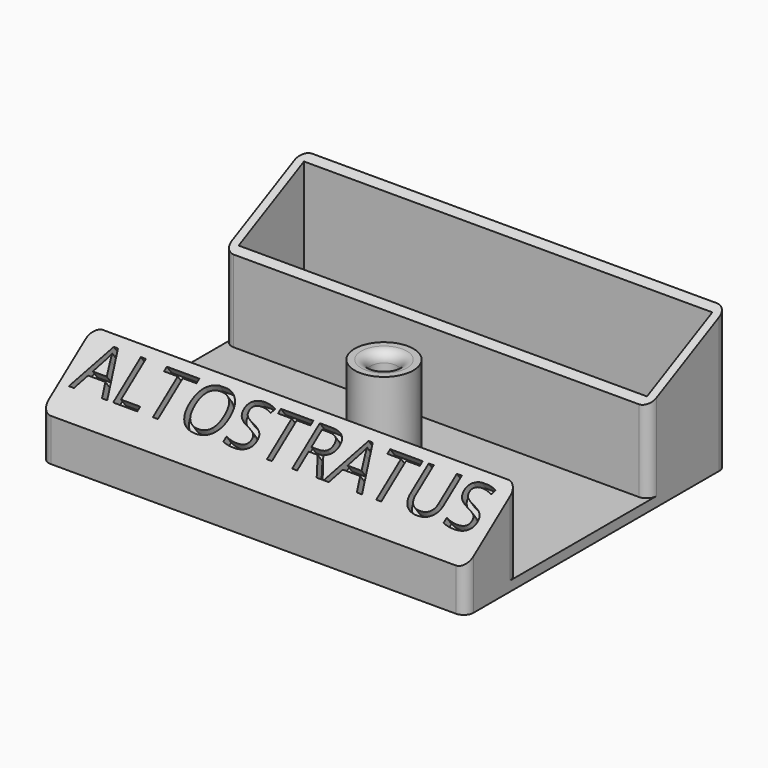
from build123d import *

# Parameters (mm, degrees)
F0_W        = 130
F0_H        = 100
F1_DEPTH    = 3
F2_W        = 130
F2_H        = 30
F2_W_2      = 125
F2_H_2      = 25
F3_DEPTH    = 40
F2_R        = 9
F2_R_2      = 4
F2_H_3      = 20
F4_DEPTH    = 25
F5_T1_DEPTH = 233.2279032045
F6_T1_DEPTH = 285.3897324272
F7_R        = 3
F9_DEPTH    = 3


# Not quite as in the source:
# - a fillet or chamfer that OpenCascade refuses, or shapes differently, is made with other operations: its cross-section is extruded or revolved along the edge and cut away or added


with BuildPart() as f1:
    # F0 (on Top) → F1 (new body)
    with BuildSketch(Plane.XY):
        with Locations((0, 50)):
            Rectangle(F0_W, F0_H)
    extrude(amount=F1_DEPTH)

    # F2 (on face) → F3 (join)
    with BuildSketch(Plane.XY.offset(3)):
        with Locations((0, 85)):
            Rectangle(F2_W, F2_H)
        with Locations((0, 85)):
            Rectangle(F2_W_2, F2_H_2, mode=Mode.SUBTRACT)
    extrude(amount=F3_DEPTH)

    # F2 (on face) → F4 (join)
    with BuildSketch(Plane.XY.offset(3)):
        with Locations((0, 50)):
            Circle(F2_R)
        with Locations((0, 50)):
            Circle(F2_R_2, mode=Mode.SUBTRACT)
        with Locations((0, 10)):
            Rectangle(F2_W, F2_H_3)
    extrude(amount=F4_DEPTH)

    # F5: chamfer of 20 x 15 on 1 edges, made by hand

    # F5_s2 → F5_t1 (cut)
    with BuildSketch(Plane.YZ.offset(-116.6139516023)):
        Polygon((0, 13), (20, 28), (0, 28), align=None)
    extrude(amount=F5_T1_DEPTH, mode=Mode.SUBTRACT)

    # F6: chamfer of 30 x 15 on 1 edges, made by hand

    # F6_s2 → F6_t1 (cut)
    with BuildSketch(Plane.YZ.offset(-142.6948662136)):
        Polygon((100, 43), (70, 28), (70, 43), align=None)
    extrude(amount=F6_T1_DEPTH, mode=Mode.SUBTRACT)

    # F7
    f7_edges = [f1.edges().sort_by_distance(p)[0] for p in [
        (-65, 100, 21.5),
        (-65, 70, 15.5),
        (65, 70, 15.5),
        (-65, 0, 6.5),
        (65, 100, 21.5),
        (65, 0, 6.5),
        (65, 20, 15.5),
        (-65, 20, 15.5),
        (-4, 50, 28),
    ]]
    fillet(f7_edges, radius=F7_R)

    # F8 (on face) → F9 (cut)
    with BuildSketch(Plane(origin=(0, -6.24, 8.32), x_dir=(1, 0, 0), z_dir=(0, -0.6, 0.8))):
        Polygon((-56.7649726495, 29.7420262752), (-62, 16.4428538034), (-60.4405068026, 16.4428538034), (-58.8114451353, 20.6546449109), (-53.5039506288, 20.6546449109), (-51.8545981579, 16.4428538034), (-50.2603207256, 16.4428538034), (-55.4692598999, 29.7420262752), align=None)
        with BuildLine():
            Line((-55.5243349385, 26.1447566506), (-53.9822338585, 22.0402169339))
            Line((-53.9822338585, 22.0402169339), (-58.2664921221, 22.0402169339))
            Line((-58.2664921221, 22.0402169339), (-56.7098976109, 26.1447566506))
            add(Edge.make_bspline(
                [(-56.1388564215, 28.0549908832), (-56.3388657721, 27.185385011), (-56.7098976109, 26.1447566506)],
                knots=[0, 0, 0, 1, 1, 1], degree=2))
            add(Edge.make_bspline(
                [(-55.5243349385, 26.1447566506), (-55.8228996213, 26.9245032493), (-56.1388564215, 28.0549908832)],
                knots=[0, 0, 0, 1, 1, 1], degree=2))
        make_face(mode=Mode.SUBTRACT)
        Polygon((-48.4399457665, 29.6869512366), (-48.4399457665, 16.4428538034), (-41.0569919117, 16.4428538034), (-41.0569919117, 17.8371218851), (-46.9007433728, 17.8371218851), (-46.9007433728, 29.6869512366), align=None)
        Polygon((-36.2741596148, 16.4428538034), (-34.734957221, 16.4428538034), (-34.734957221, 28.3187713311), (-30.5405582309, 28.3187713311), (-30.5405582309, 29.6869512366), (-40.4685586049, 29.6869512366), (-40.4685586049, 28.3187713311), (-36.2741596148, 28.3187713311), align=None)
        with BuildLine():
            Line((-21.8651905154, 29.8), (-24.3993920062, 29.8))
            add(Edge.make_bspline(
                [(-27.638973304, 28.1158632942), (-26.4142998889, 29.4830441613), (-24.3993920062, 29.8)],
                knots=[0, 0, 0, 0.7681683189, 0.7681683189, 0.7681683189], degree=2))
            add(Edge.make_bspline(
                [(-29.2332507364, 23.101136098), (-29.2332507364, 26.3360699425), (-27.638973304, 28.1158632942)],
                knots=[0, 0, 0, 1, 1, 1], degree=2))
            add(Edge.make_bspline(
                [(-27.6433213334, 18.0501753238), (-29.2332507364, 19.8401140773), (-29.2332507364, 23.101136098)],
                knots=[0, 0, 0, 1, 1, 1], degree=2))
            add(Edge.make_bspline(
                [(-23.1286175137, 16.2602365702), (-26.0533919304, 16.2602365702), (-27.6433213334, 18.0501753238)],
                knots=[0, 0, 0, 1, 1, 1], degree=2))
            add(Edge.make_bspline(
                [(-18.6588433307, 18.0820608724), (-20.2676141942, 16.2602365702), (-23.1286175137, 16.2602365702)],
                knots=[0, 0, 0, 1, 1, 1], degree=2))
            add(Edge.make_bspline(
                [(-17.0500724672, 23.0837439806), (-17.0500724672, 19.9038851746), (-18.6588433307, 18.0820608724)],
                knots=[0, 0, 0, 1, 1, 1], degree=2))
            add(Edge.make_bspline(
                [(-18.6530459582, 28.0839777456), (-17.0500724672, 26.2722988452), (-17.0500724672, 23.0837439806)],
                knots=[0, 0, 0, 1, 1, 1], degree=2))
            add(Edge.make_bspline(
                [(-21.8651905154, 29.8), (-19.8876841836, 29.4793645284), (-18.6530459582, 28.0839777456)],
                knots=[0.2297825059, 0.2297825059, 0.2297825059, 1, 1, 1], degree=2))
        make_face()
        with BuildLine():
            add(Edge.make_bspline(
                [(-27.6041890691, 23.0837439806), (-27.6041890691, 20.3937631493), (-26.457758661, 19.0023937538)],
                knots=[0, 0, 0, 1, 1, 1], degree=2))
            add(Edge.make_bspline(
                [(-26.457758661, 27.1274112862), (-27.6041890691, 25.7360418907), (-27.6041890691, 23.0837439806)],
                knots=[0, 0, 0, 1, 1, 1], degree=2))
            add(Edge.make_bspline(
                [(-23.1112253962, 28.5187806817), (-25.3113282528, 28.5187806817), (-26.457758661, 27.1274112862)],
                knots=[0, 0, 0, 1, 1, 1], degree=2))
            add(Edge.make_bspline(
                [(-19.8009257095, 27.137556688), (-20.9198185983, 28.5187806817), (-23.1112253962, 28.5187806817)],
                knots=[0, 0, 0, 1, 1, 1], degree=2))
            add(Edge.make_bspline(
                [(-18.6820328206, 23.0837439806), (-18.6820328206, 25.7563326944), (-19.8009257095, 27.137556688)],
                knots=[0, 0, 0, 1, 1, 1], degree=2))
            add(Edge.make_bspline(
                [(-19.8052737388, 18.9965963813), (-18.6820328206, 20.3821684043), (-18.6820328206, 23.0837439806)],
                knots=[0, 0, 0, 1, 1, 1], degree=2))
            add(Edge.make_bspline(
                [(-23.1286175137, 17.6110243583), (-20.9285146571, 17.6110243583), (-19.8052737388, 18.9965963813)],
                knots=[0, 0, 0, 1, 1, 1], degree=2))
            add(Edge.make_bspline(
                [(-26.457758661, 19.0023937538), (-25.3113282528, 17.6110243583), (-23.1286175137, 17.6110243583)],
                knots=[0, 0, 0, 1, 1, 1], degree=2))
        make_face(mode=Mode.SUBTRACT)
        with BuildLine():
            add(Edge.make_bspline(
                [(-9.3514638491, 29.8), (-8.0830896091, 29.6416662862), (-6.9597456637, 29.1506942821)],
                knots=[0.3224903099, 0.3224903099, 0.3224903099, 1, 1, 1], degree=2))
            Line((-9.3514638491, 29.8), (-11.6233285754, 29.8))
            add(Edge.make_bspline(
                [(-13.6368694189, 28.9695263921), (-12.819057523, 29.6140817955), (-11.6233285754, 29.8)],
                knots=[0, 0, 0, 0.711555898, 0.711555898, 0.711555898], degree=2))
            add(Edge.make_bspline(
                [(-14.7861985133, 26.5331806069), (-14.7861985133, 28.0636869419), (-13.6368694189, 28.9695263921)],
                knots=[0, 0, 0, 1, 1, 1], degree=2))
            add(Edge.make_bspline(
                [(-13.9934078265, 24.1693019777), (-14.7861985133, 25.0751414278), (-14.7861985133, 26.5331806069)],
                knots=[0, 0, 0, 1, 1, 1], degree=2))
            add(Edge.make_bspline(
                [(-11.3541540044, 22.6025620646), (-13.2006171397, 23.2634625275), (-13.9934078265, 24.1693019777)],
                knots=[0, 0, 0, 1, 1, 1], degree=2))
            add(Edge.make_bspline(
                [(-9.3844967039, 21.7604937117), (-10.0323530787, 22.1329748936), (-11.3541540044, 22.6025620646)],
                knots=[0, 0, 0, 1, 1, 1], degree=2))
            add(Edge.make_bspline(
                [(-8.4598157932, 20.9488615644), (-8.7366403291, 21.3880125298), (-9.3844967039, 21.7604937117)],
                knots=[0, 0, 0, 1, 1, 1], degree=2))
            add(Edge.make_bspline(
                [(-8.1829912572, 19.8227219599), (-8.1829912572, 20.5097105989), (-8.4598157932, 20.9488615644)],
                knots=[0, 0, 0, 1, 1, 1], degree=2))
            add(Edge.make_bspline(
                [(-8.9627378559, 18.1951096358), (-8.1829912572, 18.7791949133), (-8.1829912572, 19.8227219599)],
                knots=[0, 0, 0, 1, 1, 1], degree=2))
            add(Edge.make_bspline(
                [(-11.2816868484, 17.6110243583), (-9.7424844546, 17.6110243583), (-8.9627378559, 18.1951096358)],
                knots=[0, 0, 0, 1, 1, 1], degree=2))
            add(Edge.make_bspline(
                [(-13.1832250222, 17.8110337089), (-12.2237598766, 17.6110243583), (-11.2816868484, 17.6110243583)],
                knots=[0, 0, 0, 1, 1, 1], degree=2))
            add(Edge.make_bspline(
                [(-14.9601196877, 18.3530880359), (-14.1426901678, 18.0110430595), (-13.1832250222, 17.8110337089)],
                knots=[0, 0, 0, 1, 1, 1], degree=2))
            Line((-14.9601196877, 18.3530880359), (-14.9601196877, 16.8689606807))
            add(Edge.make_bspline(
                [(-11.336761887, 16.2602365702), (-13.6904951143, 16.2602365702), (-14.9601196877, 16.8689606807)],
                knots=[0, 0, 0, 1, 1, 1], degree=2))
            add(Edge.make_bspline(
                [(-7.8945719762, 17.2399925195), (-9.1627472065, 16.2602365702), (-11.336761887, 16.2602365702)],
                knots=[0, 0, 0, 1, 1, 1], degree=2))
            add(Edge.make_bspline(
                [(-6.626396746, 19.9676562719), (-6.626396746, 18.2197484688), (-7.8945719762, 17.2399925195)],
                knots=[0, 0, 0, 1, 1, 1], degree=2))
            add(Edge.make_bspline(
                [(-7.409042031, 22.1764551872), (-6.626396746, 21.3242414325), (-6.626396746, 19.9676562719)],
                knots=[0, 0, 0, 1, 1, 1], degree=2))
            add(Edge.make_bspline(
                [(-10.2758427229, 23.7707326196), (-8.1916873159, 23.028668942), (-7.409042031, 22.1764551872)],
                knots=[0, 0, 0, 1, 1, 1], degree=2))
            add(Edge.make_bspline(
                [(-12.1194071719, 24.5809154238), (-11.5164804339, 24.2142316144), (-10.2758427229, 23.7707326196)],
                knots=[0, 0, 0, 1, 1, 1], degree=2))
            add(Edge.make_bspline(
                [(-12.975968956, 25.3881995418), (-12.72233391, 24.9475992333), (-12.1194071719, 24.5809154238)],
                knots=[0, 0, 0, 1, 1, 1], degree=2))
            add(Edge.make_bspline(
                [(-13.2296040021, 26.5157884894), (-13.2296040021, 25.8287998504), (-12.975968956, 25.3881995418)],
                knots=[0, 0, 0, 1, 1, 1], degree=2))
            add(Edge.make_bspline(
                [(-12.5411660199, 27.9738276684), (-13.2296040021, 27.4491654589), (-13.2296040021, 26.5157884894)],
                knots=[0, 0, 0, 1, 1, 1], degree=2))
            add(Edge.make_bspline(
                [(-10.6294824442, 28.498489878), (-11.8527280378, 28.498489878), (-12.5411660199, 27.9738276684)],
                knots=[0, 0, 0, 1, 1, 1], degree=2))
            add(Edge.make_bspline(
                [(-7.4409275796, 27.811501239), (-9.0815839918, 28.498489878), (-10.6294824442, 28.498489878)],
                knots=[0, 0, 0, 1, 1, 1], degree=2))
            Line((-7.4409275796, 27.811501239), (-6.9597456637, 29.1506942821))
        make_face()
        with BuildLine():
            Line((-11.6233285754, 29.8), (-9.3514638491, 29.8))
            add(Edge.make_bspline(
                [(-10.5917995231, 29.8753658423), (-9.9552019325, 29.8753658423), (-9.3514638491, 29.8)],
                knots=[0, 0, 0, 0.3224903099, 0.3224903099, 0.3224903099], degree=2))
            add(Edge.make_bspline(
                [(-11.6233285754, 29.8), (-11.1386147763, 29.8753658423), (-10.5917995231, 29.8753658423)],
                knots=[0.711555898, 0.711555898, 0.711555898, 1, 1, 1], degree=2))
        make_face()
        Polygon((-1.3797746505, 16.4428538034), (0.1594277432, 16.4428538034), (0.1594277432, 28.3187713311), (4.3538267334, 28.3187713311), (4.3538267334, 29.6869512366), (-5.5741736407, 29.6869512366), (-5.5741736407, 28.3187713311), (-1.3797746505, 28.3187713311), align=None)
        with BuildLine():
            Line((7.8873252606, 16.4428538034), (7.8873252606, 21.9503576605))
            Line((7.8873252606, 21.9503576605), (10.6526719342, 21.9503576605))
            Line((10.6526719342, 21.9503576605), (13.8586189163, 16.4428538034))
            Line((13.8586189163, 16.4428538034), (15.6789938754, 16.4428538034))
            Line((15.6789938754, 16.4428538034), (12.0817242508, 22.3938566553))
            add(Edge.make_bspline(
                [(14.7456169059, 25.9447473), (14.7456169059, 23.318537566), (12.0817242508, 22.3938566553)],
                knots=[0, 0, 0, 1, 1, 1], degree=2))
            add(Edge.make_bspline(
                [(13.5817943803, 28.7535742671), (14.7456169059, 27.8201972977), (14.7456169059, 25.9447473)],
                knots=[0, 0, 0, 1, 1, 1], degree=2))
            add(Edge.make_bspline(
                [(9.9801767264, 29.6869512366), (12.4179718547, 29.6869512366), (13.5817943803, 28.7535742671)],
                knots=[0, 0, 0, 1, 1, 1], degree=2))
            Line((9.9801767264, 29.6869512366), (6.3481228669, 29.6869512366))
            Line((6.3481228669, 29.6869512366), (6.3481228669, 16.4428538034))
            Line((6.3481228669, 16.4428538034), (7.8873252606, 16.4428538034))
        make_face()
        with BuildLine():
            Line((10.00046753, 23.2721585862), (7.8873252606, 23.2721585862))
            Line((7.8873252606, 23.2721585862), (7.8873252606, 28.3361634485))
            Line((7.8873252606, 28.3361634485), (9.8903174529, 28.3361634485))
            add(Edge.make_bspline(
                [(12.3773902473, 27.7564262004), (11.6034410211, 28.3361634485), (9.8903174529, 28.3361634485)],
                knots=[0, 0, 0, 1, 1, 1], degree=2))
            add(Edge.make_bspline(
                [(13.1513394736, 25.8635840853), (13.1513394736, 27.1766889523), (12.3773902473, 27.7564262004)],
                knots=[0, 0, 0, 1, 1, 1], degree=2))
            add(Edge.make_bspline(
                [(12.3904343354, 23.920014961), (13.1513394736, 24.5678713357), (13.1513394736, 25.8635840853)],
                knots=[0, 0, 0, 1, 1, 1], degree=2))
            add(Edge.make_bspline(
                [(10.00046753, 23.2721585862), (11.6295291973, 23.2721585862), (12.3904343354, 23.920014961)],
                knots=[0, 0, 0, 1, 1, 1], degree=2))
        make_face(mode=Mode.SUBTRACT)
        Polygon((24.4910000468, 20.6546449109), (26.1403525176, 16.4428538034), (27.73462995, 16.4428538034), (22.5256907756, 29.7420262752), (21.2299780261, 29.7420262752), (15.9949506756, 16.4428538034), (17.554443873, 16.4428538034), (19.1835055402, 20.6546449109), align=None)
        with BuildLine():
            Line((22.4706157371, 26.1447566506), (24.0127168171, 22.0402169339))
            Line((24.0127168171, 22.0402169339), (19.7284585535, 22.0402169339))
            Line((19.7284585535, 22.0402169339), (21.2850530647, 26.1447566506))
            add(Edge.make_bspline(
                [(21.8560942541, 28.0549908832), (21.6560849035, 27.185385011), (21.2850530647, 26.1447566506)],
                knots=[0, 0, 0, 1, 1, 1], degree=2))
            add(Edge.make_bspline(
                [(22.4706157371, 26.1447566506), (22.1720510543, 26.9245032493), (21.8560942541, 28.0549908832)],
                knots=[0, 0, 0, 1, 1, 1], degree=2))
        make_face(mode=Mode.SUBTRACT)
        Polygon((32.0913553696, 16.4428538034), (33.6305577633, 16.4428538034), (33.6305577633, 28.3187713311), (37.8249567535, 28.3187713311), (37.8249567535, 29.6869512366), (27.8969563794, 29.6869512366), (27.8969563794, 28.3187713311), (32.0913553696, 28.3187713311), align=None)
        with BuildLine():
            Line((49.819720417, 21.1184347094), (49.819720417, 29.6869512366))
            Line((49.819720417, 29.6869512366), (48.2805180233, 29.6869512366))
            Line((48.2805180233, 29.6869512366), (48.2805180233, 21.0633596709))
            add(Edge.make_bspline(
                [(47.3746785731, 18.5038197204), (48.2805180233, 19.3966150825), (48.2805180233, 21.0633596709)],
                knots=[0, 0, 0, 1, 1, 1], degree=2))
            add(Edge.make_bspline(
                [(44.7933984759, 17.6110243583), (46.4688391229, 17.6110243583), (47.3746785731, 18.5038197204)],
                knots=[0, 0, 0, 1, 1, 1], degree=2))
            add(Edge.make_bspline(
                [(42.1309551639, 18.4994716911), (43.0367946141, 17.6110243583), (44.7933984759, 17.6110243583)],
                knots=[0, 0, 0, 1, 1, 1], degree=2))
            add(Edge.make_bspline(
                [(41.2251157137, 21.0459675534), (41.2251157137, 19.3879190238), (42.1309551639, 18.4994716911)],
                knots=[0, 0, 0, 1, 1, 1], degree=2))
            Line((41.2251157137, 21.0459675534), (41.2251157137, 29.6869512366))
            Line((41.2251157137, 29.6869512366), (39.6830146337, 29.6869512366))
            Line((39.6830146337, 29.6869512366), (39.6830146337, 21.1532189443))
            add(Edge.make_bspline(
                [(40.9917714713, 17.5660947216), (39.6830146337, 18.871952873), (39.6830146337, 21.1532189443)],
                knots=[0, 0, 0, 1, 1, 1], degree=2))
            add(Edge.make_bspline(
                [(44.6919444574, 16.2602365702), (42.3005283089, 16.2602365702), (40.9917714713, 17.5660947216)],
                knots=[0, 0, 0, 1, 1, 1], degree=2))
            add(Edge.make_bspline(
                [(48.4515405115, 17.5559493197), (47.0833606059, 16.2602365702), (44.6919444574, 16.2602365702)],
                knots=[0, 0, 0, 1, 1, 1], degree=2))
            add(Edge.make_bspline(
                [(49.819720417, 21.1184347094), (49.819720417, 18.8516620693), (48.4515405115, 17.5559493197)],
                knots=[0, 0, 0, 1, 1, 1], degree=2))
        make_face()
        with BuildLine():
            add(Edge.make_bspline(
                [(58.0719781071, 29.8), (59.3403523471, 29.6416662862), (60.4636962925, 29.1506942821)],
                knots=[0.3224903099, 0.3224903099, 0.3224903099, 1, 1, 1], degree=2))
            Line((58.0719781071, 29.8), (55.8001133808, 29.8))
            add(Edge.make_bspline(
                [(53.7865725373, 28.9695263921), (54.6043844331, 29.6140817955), (55.8001133808, 29.8)],
                knots=[0, 0, 0, 0.711555898, 0.711555898, 0.711555898], degree=2))
            add(Edge.make_bspline(
                [(52.6372434429, 26.5331806069), (52.6372434429, 28.0636869419), (53.7865725373, 28.9695263921)],
                knots=[0, 0, 0, 1, 1, 1], degree=2))
            add(Edge.make_bspline(
                [(53.4300341297, 24.1693019777), (52.6372434429, 25.0751414278), (52.6372434429, 26.5331806069)],
                knots=[0, 0, 0, 1, 1, 1], degree=2))
            add(Edge.make_bspline(
                [(56.0692879518, 22.6025620646), (54.2228248165, 23.2634625275), (53.4300341297, 24.1693019777)],
                knots=[0, 0, 0, 1, 1, 1], degree=2))
            add(Edge.make_bspline(
                [(58.0389452522, 21.7604937117), (57.3910888775, 22.1329748936), (56.0692879518, 22.6025620646)],
                knots=[0, 0, 0, 1, 1, 1], degree=2))
            add(Edge.make_bspline(
                [(58.963626163, 20.9488615644), (58.686801627, 21.3880125298), (58.0389452522, 21.7604937117)],
                knots=[0, 0, 0, 1, 1, 1], degree=2))
            add(Edge.make_bspline(
                [(59.240450699, 19.8227219599), (59.240450699, 20.5097105989), (58.963626163, 20.9488615644)],
                knots=[0, 0, 0, 1, 1, 1], degree=2))
            add(Edge.make_bspline(
                [(58.4607041002, 18.1951096358), (59.240450699, 18.7791949133), (59.240450699, 19.8227219599)],
                knots=[0, 0, 0, 1, 1, 1], degree=2))
            add(Edge.make_bspline(
                [(56.1417551078, 17.6110243583), (57.6809575015, 17.6110243583), (58.4607041002, 18.1951096358)],
                knots=[0, 0, 0, 1, 1, 1], degree=2))
            add(Edge.make_bspline(
                [(54.2402169339, 17.8110337089), (55.1996820796, 17.6110243583), (56.1417551078, 17.6110243583)],
                knots=[0, 0, 0, 1, 1, 1], degree=2))
            add(Edge.make_bspline(
                [(52.4633222685, 18.3530880359), (53.2807517883, 18.0110430595), (54.2402169339, 17.8110337089)],
                knots=[0, 0, 0, 1, 1, 1], degree=2))
            Line((52.4633222685, 18.3530880359), (52.4633222685, 16.8689606807))
            add(Edge.make_bspline(
                [(56.0866800692, 16.2602365702), (53.7329468418, 16.2602365702), (52.4633222685, 16.8689606807)],
                knots=[0, 0, 0, 1, 1, 1], degree=2))
            add(Edge.make_bspline(
                [(59.5288699799, 17.2399925195), (58.2606947496, 16.2602365702), (56.0866800692, 16.2602365702)],
                knots=[0, 0, 0, 1, 1, 1], degree=2))
            add(Edge.make_bspline(
                [(60.7970452102, 19.9676562719), (60.7970452102, 18.2197484688), (59.5288699799, 17.2399925195)],
                knots=[0, 0, 0, 1, 1, 1], degree=2))
            add(Edge.make_bspline(
                [(60.0143999252, 22.1764551872), (60.7970452102, 21.3242414325), (60.7970452102, 19.9676562719)],
                knots=[0, 0, 0, 1, 1, 1], degree=2))
            add(Edge.make_bspline(
                [(57.1475992333, 23.7707326196), (59.2317546402, 23.028668942), (60.0143999252, 22.1764551872)],
                knots=[0, 0, 0, 1, 1, 1], degree=2))
            add(Edge.make_bspline(
                [(55.3040347842, 24.5809154238), (55.9069615223, 24.2142316144), (57.1475992333, 23.7707326196)],
                knots=[0, 0, 0, 1, 1, 1], degree=2))
            add(Edge.make_bspline(
                [(54.4474730001, 25.3881995418), (54.7011080462, 24.9475992333), (55.3040347842, 24.5809154238)],
                knots=[0, 0, 0, 1, 1, 1], degree=2))
            add(Edge.make_bspline(
                [(54.1938379541, 26.5157884894), (54.1938379541, 25.8287998504), (54.4474730001, 25.3881995418)],
                knots=[0, 0, 0, 1, 1, 1], degree=2))
            add(Edge.make_bspline(
                [(54.8822759362, 27.9738276684), (54.1938379541, 27.4491654589), (54.1938379541, 26.5157884894)],
                knots=[0, 0, 0, 1, 1, 1], degree=2))
            add(Edge.make_bspline(
                [(56.7939595119, 28.498489878), (55.5707139184, 28.498489878), (54.8822759362, 27.9738276684)],
                knots=[0, 0, 0, 1, 1, 1], degree=2))
            add(Edge.make_bspline(
                [(59.9825143765, 27.811501239), (58.3418579644, 28.498489878), (56.7939595119, 28.498489878)],
                knots=[0, 0, 0, 1, 1, 1], degree=2))
            Line((59.9825143765, 27.811501239), (60.4636962925, 29.1506942821))
        make_face()
    extrude(amount=-F9_DEPTH, mode=Mode.SUBTRACT)


solid = f1.part
